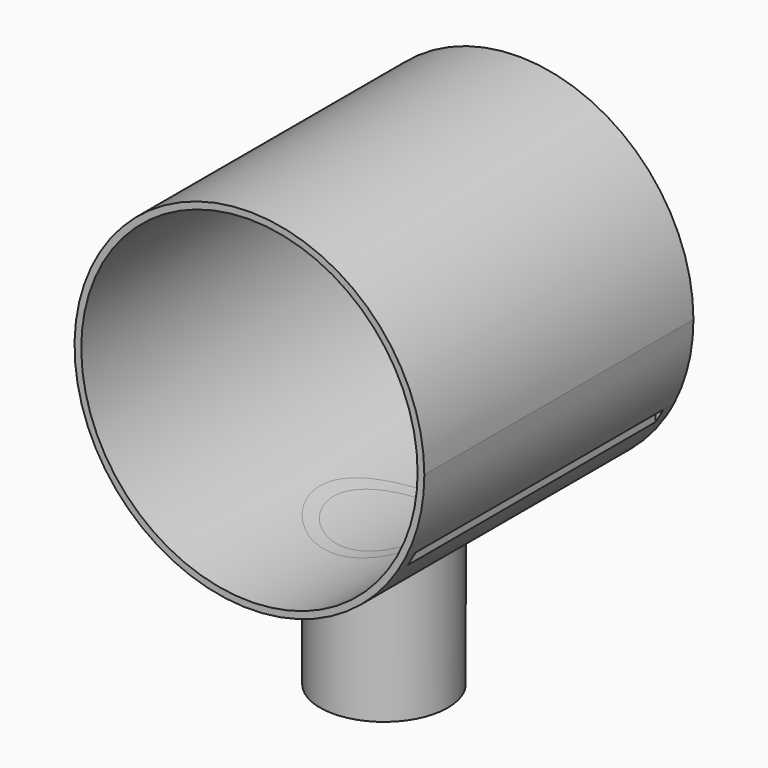
from build123d import *
from build123d import SkipClean  # not in build123d's __all__

# Parameters (mm, degrees)
F1_DEPTH = 2
F2_DEPTH = 50
F3_R     = 9.5
F3_R_2   = 7.5
F4_DEPTH = 5
F5_DEPTH = 20
F6_DEPTH = 60
F8_DEPTH = 2


# Not quite as in the source:
# - a feature names something its author has since deleted; it is built from what else it names


with BuildPart() as f1:
    # F0 (on Front) → F1 (new body)
    with BuildSketch(Plane.XZ):
        with BuildLine():
            Line((21.9700236311, 14.0702866067), (21.9700236311, 12.0961134337))
            ThreePointArc((21.9700236311, 12.0961134337), (22.5646192045, 13.0834230481), (23.1148758296, 14.0961134337))
            Line((23.1148758296, 14.0961134337), (23.1148758296, 16.4762131806))
            ThreePointArc((23.1148758296, 16.4762131806), (22.5745245911, 15.2579871773), (21.9700236311, 14.0702866067))
        make_face()
        with BuildLine():
            ThreePointArc((25, 26), (-24.2306684883, 32.1542428138), (21.9700236311, 14.0702866067))
            ThreePointArc((21.9700236311, 14.0702866067), (22.5745245911, 15.2579871773), (23.1148758296, 16.4762131806))
            ThreePointArc((23.1148758296, 16.4762131806), (24.5241910747, 21.1457181654), (25, 26))
        make_face()
    extrude(amount=F1_DEPTH)

    # F0 (on Front) → F2 (join)
    with BuildSketch(Plane.XZ):
        with BuildLine():
            ThreePointArc((23.1148758296, 14.0961134337), (25.2684266583, 19.8757356184), (26, 26))
            ThreePointArc((26, 26), (-24.9721906769, 33.2380724503), (21.9700236311, 12.0961134337))
            Line((21.9700236311, 12.0961134337), (21.9700236311, 14.0702866067))
            ThreePointArc((21.9700236311, 14.0702866067), (-24.2306684883, 32.1542428138), (25, 26))
            ThreePointArc((25, 26), (24.5241910747, 21.1457181654), (23.1148758296, 16.4762131806))
            Line((23.1148758296, 16.4762131806), (23.1148758296, 14.0961134337))
        make_face()
    extrude(amount=F2_DEPTH)

    # F3 (on Top) → F4 (join)
    with BuildSketch(Plane.XY):
        with Locations((0, -25)):
            Circle(F3_R)
        with Locations((0, -25)):
            Circle(F3_R_2, mode=Mode.SUBTRACT)
    with SkipClean():  # cleaning this boolean's faces spoils the solid; the shape is the same uncleaned
        extrude(amount=F4_DEPTH)

    # F3 (on Top) → F5 (join)
    with BuildSketch(Plane.XY):
        with Locations((0, -25)):
            Circle(F3_R)
        with Locations((0, -25)):
            Circle(F3_R_2, mode=Mode.SUBTRACT)
    extrude(amount=-F5_DEPTH)

    # F6 (cut): a face of the model
    f6_faces = [f1.faces().sort_by_distance(p)[0] for p in [
        (0.0283286742, -2, 25.9851504248),
    ]]
    extrude(f6_faces, amount=F6_DEPTH, mode=Mode.SUBTRACT)

    # F7 (on face) → F8 (join)
    with BuildSketch(Plane.XZ.offset(50)):
        Polygon((23.1148758296, 16.4762131806), (21.9700236311, 14.0702866067), (21.9700236311, 12.0961134337), (23.1148758296, 14.0961134337), align=None)
    extrude(amount=-F8_DEPTH)


solid = f1.part
